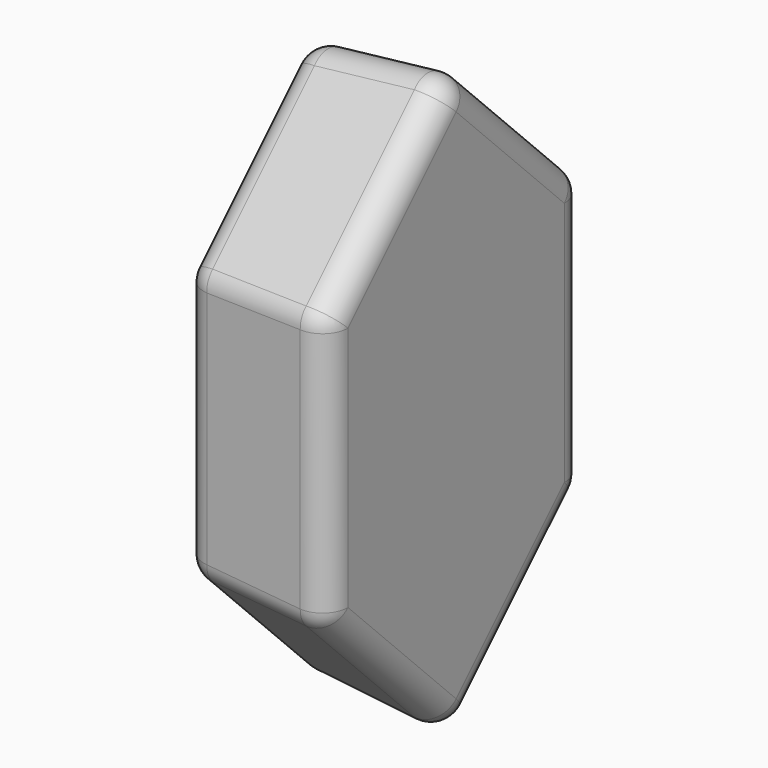
from build123d import *

# Parameters (mm, degrees)
F1_DEPTH               = 20
DRAFT_F1_DRAFTED_ANGLE = -4.583662361
F2_R                   = 3.373028188
F3_T                   = -2.5


# Not quite as in the source:
# - an extrude with a draft is written as a straight extrude whose walls are then drafted
# - a shell that OpenCascade refuses in one call is made with other operations: the cavity is built on its own and cut out


with BuildPart() as f1:
    # F0 (on Right) → F1 (new body)
    with BuildSketch(Plane.YZ):
        Polygon((0, 37.1900823038), (-20, 17.1682462096), (-20, -17.1682462096), (0, -37.1900823038), align=None)
        Polygon((20, 17.1682462096), (0, 37.1900823038), (0, -37.1900823038), (20, -17.1682462096), align=None)
    extrude(amount=F1_DEPTH)

    # draft_F1_drafted
    draft_f1_drafted_walls = [f1.faces().sort_by_distance(p)[0] for p in [
        (13.3333333333, -10, 27.1791642567),
        (13.3333333333, -20, 0),
        (13.3333333333, -10, -27.1791642567),
        (13.3333333333, 10, -27.1791642567),
        (13.3333333333, 20, 0),
        (13.3333333333, 10, 27.1791642567),
    ]]
    draft(draft_f1_drafted_walls, neutral_plane=Plane.YZ, angle=DRAFT_F1_DRAFTED_ANGLE)

    # F2
    f2_edges = [f1.edges().sort_by_distance(p)[0] for p in [
        (0, -10, 27.179164),
        (20, -10.801711, 28.645397),
        (20, -21.603422, 0),
        (20, -10.801711, -28.645397),
        (20, 10.801711, -28.645397),
        (20, 21.603422, 0),
        (20, 10.801711, 28.645397),
        (0, -20, 0),
        (0, -10, -27.179164),
        (0, 10, -27.179164),
        (0, 20, 0),
        (0, 10, 27.179164),
        (10, 0, 38.324492),
        (10, -20.801711, 17.50007),
        (10, -20.801711, -17.50007),
        (10, 0, -38.324492),
        (10, 20.801711, -17.50007),
        (10, 20.801711, 17.50007),
    ]]
    fillet(f2_edges, radius=F2_R)

    # F3: a shell. OpenCascade refuses it in one call, so the cavity is built on its own and cut out:
    # the body offset inwards by the wall thickness, plus a prism from it out through each open face.
    f3_core = offset(f1.part, amount=F3_T, mode=Mode.PRIVATE)
    f3_exits = [f3_core.faces().sort_by_distance(p)[0] for p in [
        (2.5, 0, 0),
    ]]
    add(f3_core, mode=Mode.SUBTRACT)
    extrude(f3_exits, amount=-F3_T, mode=Mode.SUBTRACT)


solid = f1.part
